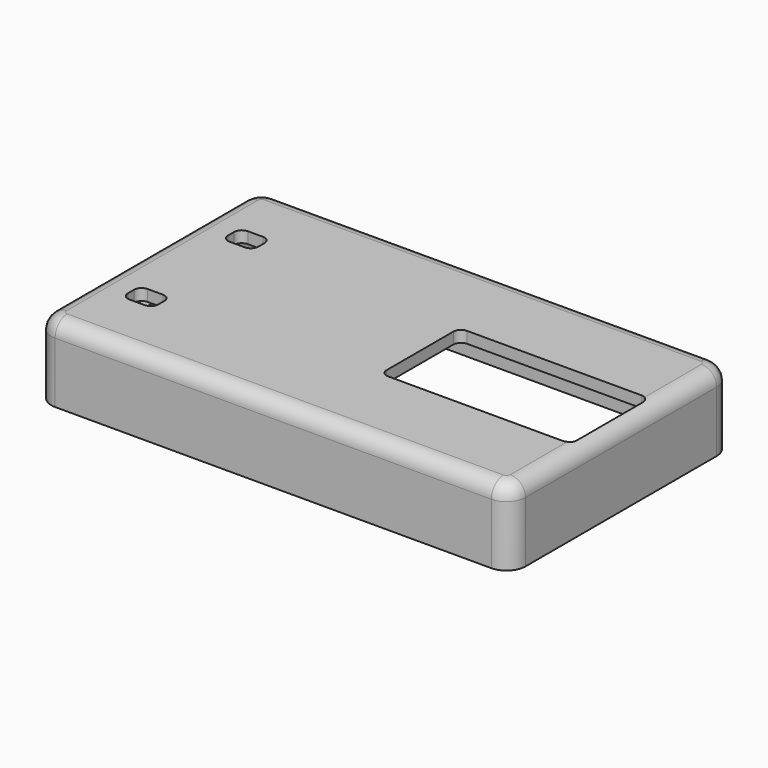
from build123d import *

# Parameters (mm, degrees)
F0_W          = 62.5
F0_H          = 36.5
F0_W_2        = 58.5
F0_H_2        = 31.5
F1_DEPTH      = 7
F2_W          = 4
F2_H          = 3
F3_DEPTH      = 1.5
F4_W          = 62.5
F4_H          = 36.5
F5_DEPTH      = 3
F7_DEPTH      = 2.5
F8_R          = 2.5
F9_R          = 1
F10_R         = 1
F11_T1_DEPTH  = 57.5
F11_T3_DEPTH  = 31.5
F11_T6_ANGLE  = 90
F11_T8_ANGLE  = 90
F11_T10_ANGLE = 90
F11_T12_ANGLE = 90
F12_W         = 1.25
F12_H         = 8.5
F13_DEPTH     = 2


# Not quite as in the source:
# - a fillet or chamfer that OpenCascade refuses, or shapes differently, is made with other operations: its cross-section is extruded or revolved along the edge and cut away or added


with BuildPart() as f1:
    # F0 (on Top) → F1 (new body)
    with BuildSketch(Plane.XY):
        with Locations((0.5, 0.5)):
            Rectangle(F0_W, F0_H)
        with Locations((1, 0.5)):
            Rectangle(F0_W_2, F0_H_2, mode=Mode.SUBTRACT)
    extrude(amount=F1_DEPTH)

    # F2 (on face) → F3 (join)
    with BuildSketch(Plane.XY.offset(7)):
        Polygon((30.25, 16.25), (-28.25, 16.25), (-28.25, -15.25), (30.25, -15.25), (30.25, -6), (5.25, -6), (5.25, 7), (30.25, 7), align=None)
        with Locations((-24.25, -7.75)):
            Rectangle(F2_W, F2_H, mode=Mode.SUBTRACT)
        with Locations((-24.25, 8.75)):
            Rectangle(F2_W, F2_H, mode=Mode.SUBTRACT)
    extrude(amount=-F3_DEPTH)

    # F4 (on face) → F5 (join)
    with BuildSketch(Plane(origin=(0, 0, 0), x_dir=(1, 0, 0), z_dir=(0, 0, -1))):
        with Locations((0.5, -0.5)):
            Rectangle(F4_W, F4_H)
        Polygon((-29.5, -17.522141248), (-29.5, 16.5), (30.25, 16.5), (30.25, 15.25), (30.25, -16.25), (30.25, -17.522141248), align=None, mode=Mode.SUBTRACT)
    extrude(amount=F5_DEPTH)

    # F6 (on face) → F7 (cut)
    with BuildSketch(Plane.YZ.offset(-28.25)):
        with BuildLine():
            Line((4, 5.5), (-3, 5.5))
            ThreePointArc((-3, 5.5), (-3.5303300859, 5.2803300859), (-3.75, 4.75))
            Line((-3.75, 4.75), (-3.75, 3.5))
            ThreePointArc((-3.75, 3.5), (-3.1642135624, 2.0857864376), (-1.75, 1.5))
            Line((-1.75, 1.5), (2.75, 1.5))
            ThreePointArc((2.75, 1.5), (4.1642135624, 2.0857864376), (4.75, 3.5))
            Line((4.75, 3.5), (4.75, 4.75))
            ThreePointArc((4.75, 4.75), (4.5303300859, 5.2803300859), (4, 5.5))
        make_face()
    extrude(amount=-F7_DEPTH, mode=Mode.SUBTRACT)

    # F8
    f8_edges = [f1.edges().sort_by_distance(p)[0] for p in [
        (-30.75, 18.75, 2),
        (-30.75, -17.75, 2),
        (31.75, 18.75, 2),
        (31.75, -17.75, 2),
    ]]
    fillet(f8_edges, radius=F8_R)

    # F9
    f9_edges = [f1.edges().sort_by_distance(p)[0] for p in [
        (5.25, 7, 6.25),
        (30.25, 7, 6.25),
        (30.25, -6, 6.25),
        (5.25, -6, 6.25),
    ]]
    fillet(f9_edges, radius=F9_R)

    # F10
    f10_edges = [f1.edges().sort_by_distance(p)[0] for p in [
        (-22.25, 10.25, 6.25),
        (-26.25, 10.25, 6.25),
        (-26.25, 7.25, 6.25),
        (-22.25, 7.25, 6.25),
        (-26.25, -6.25, 6.25),
        (-22.25, -6.25, 6.25),
        (-22.25, -9.25, 6.25),
        (-26.25, -9.25, 6.25),
    ]]
    fillet(f10_edges, radius=F10_R)

    # F11: fillet of radius 2 on 8 edges, made by hand

    # F11_s2 → F11_t1 (cut)
    with BuildSketch(Plane.YZ.offset(-28.25)):
        with BuildLine():
            ThreePointArc((-15.75, 7), (-17.1642135624, 6.4142135624), (-17.75, 5))
            Line((-17.75, 5), (-17.75, 7))
            Line((-17.75, 7), (-15.75, 7))
        make_face()
        with BuildLine():
            ThreePointArc((16.75, 7), (18.1642135624, 6.4142135624), (18.75, 5))
            Line((18.75, 5), (18.75, 7))
            Line((18.75, 7), (16.75, 7))
        make_face()
    extrude(amount=F11_T1_DEPTH, mode=Mode.SUBTRACT)

    # F11_s4 → F11_t3 (cut)
    with BuildSketch(Plane.XZ.offset(-16.25)):
        with BuildLine():
            ThreePointArc((29.75, 7), (31.1642135624, 6.4142135624), (31.75, 5))
            Line((31.75, 5), (31.75, 7))
            Line((31.75, 7), (29.75, 7))
        make_face()
        with BuildLine():
            ThreePointArc((-28.75, 7), (-30.1642135624, 6.4142135624), (-30.75, 5))
            Line((-30.75, 5), (-30.75, 7))
            Line((-30.75, 7), (-28.75, 7))
        make_face()
    extrude(amount=F11_T3_DEPTH, mode=Mode.SUBTRACT)

    # F11_s5 → F11_t6 (revolve, cut)
    with BuildSketch(Plane.YZ.offset(29.25)):
        with BuildLine():
            ThreePointArc((16.75, 7), (18.1642135624, 6.4142135624), (18.75, 5))
            Line((18.75, 5), (18.75, 7))
            Line((18.75, 7), (16.75, 7))
        make_face()
    revolve(axis=Axis((29.25, 16.25, 7), (0, 0, -1)), revolution_arc=F11_T6_ANGLE, mode=Mode.SUBTRACT)

    # F11_s7 → F11_t8 (revolve, cut)
    with BuildSketch(Plane.YZ.offset(-28.25)):
        with BuildLine():
            ThreePointArc((16.75, 7), (18.1642135624, 6.4142135624), (18.75, 5))
            Line((18.75, 5), (18.75, 7))
            Line((18.75, 7), (16.75, 7))
        make_face()
    revolve(axis=Axis((-28.25, 16.25, 7), (0, 0, 1)), revolution_arc=F11_T8_ANGLE, mode=Mode.SUBTRACT)

    # F11_s9 → F11_t10 (revolve, cut)
    with BuildSketch(Plane.XZ.offset(15.25)):
        with BuildLine():
            ThreePointArc((29.75, 7), (31.1642135624, 6.4142135624), (31.75, 5))
            Line((31.75, 5), (31.75, 7))
            Line((31.75, 7), (29.75, 7))
        make_face()
    revolve(axis=Axis((29.25, -15.25, 7), (0, 0, -1)), revolution_arc=F11_T10_ANGLE, mode=Mode.SUBTRACT)

    # F11_s11 → F11_t12 (revolve, cut)
    with BuildSketch(Plane.XZ.offset(15.25)):
        with BuildLine():
            ThreePointArc((-28.75, 7), (-30.1642135624, 6.4142135624), (-30.75, 5))
            Line((-30.75, 5), (-30.75, 7))
            Line((-30.75, 7), (-28.75, 7))
        make_face()
    revolve(axis=Axis((-28.25, -15.25, 7), (0, 0, 1)), revolution_arc=F11_T12_ANGLE, mode=Mode.SUBTRACT)

    # F12 (on face) → F13 (cut)
    with BuildSketch(Plane(origin=(0, 0, 0), x_dir=(1, 0, 0), z_dir=(0, 0, -1))):
        with Locations((-28.875, -0.5)):
            Rectangle(F12_W, F12_H)
    extrude(amount=-F13_DEPTH, mode=Mode.SUBTRACT)


solid = f1.part
